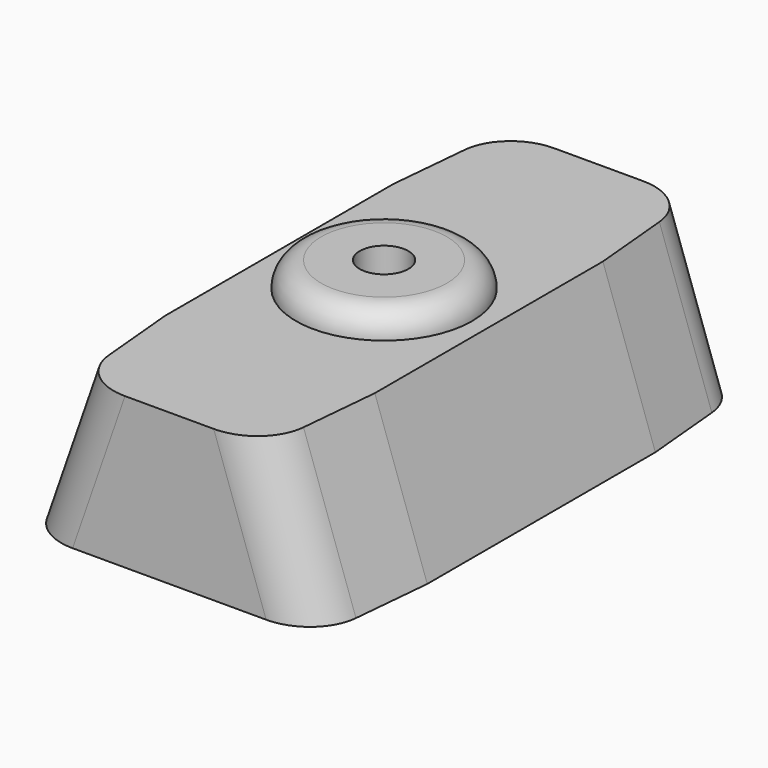
from build123d import *

# Parameters (mm, degrees)
F1_DEPTH   = 16
F2_R       = 5.25
F3_DEPTH   = 1.5
F4_R       = 1.45
F5_DEPTH   = 12
F6_SIZE2   = 0.6561649764
F6_SIZE    = 7.5
F6_2_SIZE2 = 0.6561649764
F6_2_SIZE  = 7.5
F7_R       = 3
F8_R       = 1.49999


# Not quite as in the source:
# - a fillet or chamfer is up to 0.001 mm smaller than in the source, because OpenCascade refuses the exact size


with BuildPart() as f1:
    # F0 (on Front) → F1 (new body, symmetric)
    with BuildSketch(Plane.XZ):
        Polygon((6.25, 0), (0, 0), (-6.25, 0), (-9.375, -9), (0, -9), (9.375, -9), align=None)
    extrude(amount=F1_DEPTH, both=True)

    # F2 (on face) → F3 (join)
    with BuildSketch(Plane.XY):
        Circle(F2_R)
    extrude(amount=F3_DEPTH)

    # F4 (on face) → F5 (cut)
    with BuildSketch(Plane.XY.offset(1.5)):
        Circle(F4_R)
    extrude(amount=-F5_DEPTH, mode=Mode.SUBTRACT)

    # F6
    f6_edges = [f1.edges().sort_by_distance(p)[0] for p in [
        (7.8125, -16, -4.5),
        (7.8125, 16, -4.5),
    ]]
    f6_side = f1.faces().sort_by_distance((7.8125, 0, -4.5))[0]
    chamfer(f6_edges, length=F6_SIZE, length2=F6_SIZE2, reference=f6_side)

    # F6#2
    f6_2_edges = [f1.edges().sort_by_distance(p)[0] for p in [
        (-7.8125, -16, -4.5),
        (-7.8125, 16, -4.5),
    ]]
    f6_2_side = f1.faces().sort_by_distance((-7.8125, 0, -4.5))[0]
    chamfer(f6_2_edges, length=F6_2_SIZE, length2=F6_2_SIZE2, reference=f6_2_side)

    # F7
    f7_edges = [f1.edges().sort_by_distance(p)[0] for p in [
        (7.117906, -16, -4.5),
        (-7.117906, -16, -4.5),
        (7.117906, 16, -4.5),
        (-7.117906, 16, -4.5),
    ]]
    fillet(f7_edges, radius=F7_R)

    # F8 (radius 1.5 in the source; OpenCascade refuses exactly that, so slightly less here)
    f8_edges = [f1.edges().sort_by_distance(p)[0] for p in [
        (-5.25, 0, 1.5),
    ]]
    fillet(f8_edges, radius=F8_R)


solid = f1.part
